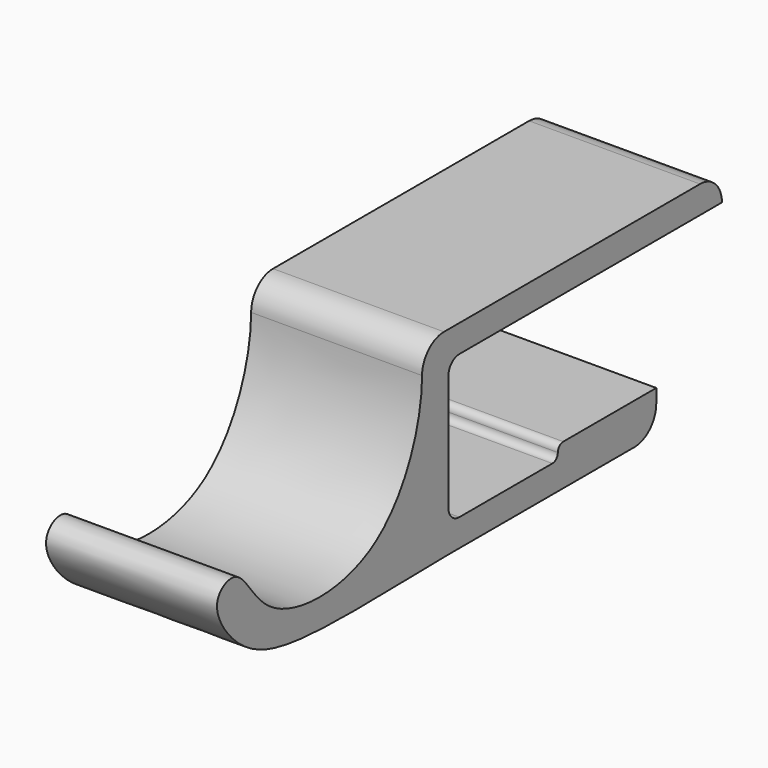
from build123d import *

# Parameters (mm, degrees)
F1_DEPTH = 25
F2_R     = 3.99999
F3_R     = 2
F4_W     = 25
F4_H     = 18
F5_DEPTH = 2
F6_R     = 0.99999


# Not quite as in the source:
# - a fillet or chamfer is up to 0.001 mm smaller than in the source, because OpenCascade refuses the exact size


with BuildPart() as f1:
    # F0 (on Right) → F1 (new body)
    with BuildSketch(Plane.YZ):
        with BuildLine():
            Line((38, -4), (38, 0))
            Line((38, 0), (0, 0))
            Line((0, 0), (0, 21))
            Line((0, 21), (50, 21))
            Line((50, 21), (50, 25))
            Line((50, 25), (-4.8117317967, 25))
            Line((-4.8117317967, 25), (-4.8117317967, 21))
            add(Edge.make_bspline(
                [(-4.8117317967, 21), (-4.8117317967, 15.1116313237), (-10.4022162379, -1.2338685341), (-33.9842886789, -0.4463867162), (-37.7851196704, 10.6094730484), (-44.1713858953, 7.385774766), (-38.045766604, -1.9056337415), (-25.67183797, -4.930685629), (-6.9570716316, -4), (0, -4)],
                knots=[0, 0, 0, 0, 0.1769849674, 0.3491823831, 0.4679710597, 0.5431517863, 0.6569534494, 0.8005937823, 1, 1, 1, 1], degree=3))
            Line((0, -4), (38, -4))
        make_face()
    extrude(amount=F1_DEPTH)

    # F2 (radius 4 in the source; OpenCascade refuses exactly that, so slightly less here)
    f2_edges = [f1.edges().sort_by_distance(p)[0] for p in [
        (12.5, -4.811732, 25),
        (12.5, 50, 25),
        (12.5, 38, -4),
    ]]
    fillet(f2_edges, radius=F2_R)

    # F3
    f3_edges = [f1.edges().sort_by_distance(p)[0] for p in [
        (12.5, 0, 21),
        (12.5, 0, 0),
    ]]
    fillet(f3_edges, radius=F3_R)

    # F4 (on face) → F5 (join)
    with BuildSketch(Plane.XY):
        with Locations((12.5, 29)):
            Rectangle(F4_W, F4_H)
    extrude(amount=F5_DEPTH)

    # F6 (radius 1 in the source; OpenCascade refuses exactly that, so slightly less here)
    f6_edges = [f1.edges().sort_by_distance(p)[0] for p in [
        (12.5, 20, 0),
        (12.5, 20, 2),
    ]]
    fillet(f6_edges, radius=F6_R)


solid = f1.part
